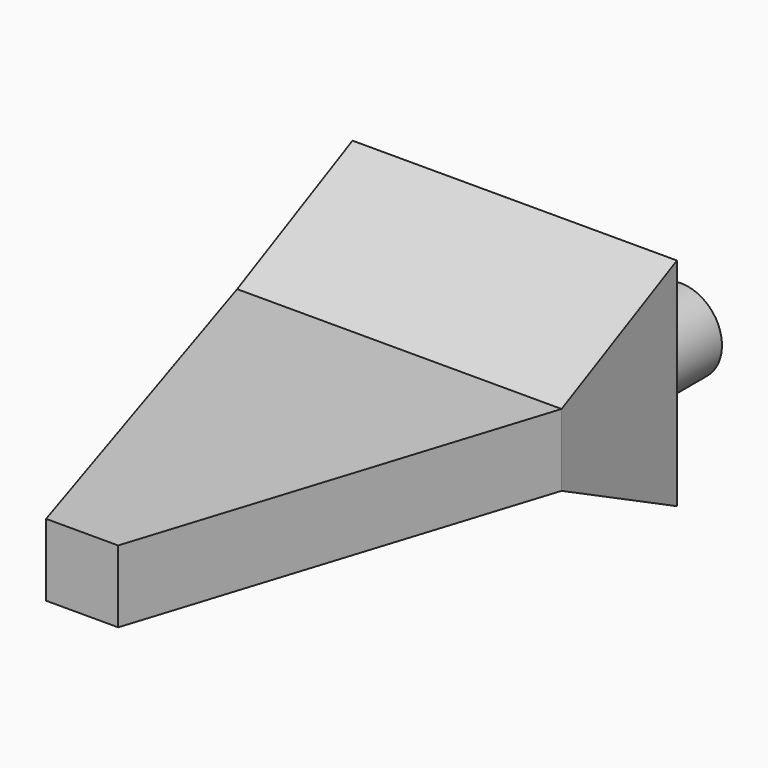
from build123d import *

# Parameters (mm, degrees)
F0_W          = 9
F0_H          = 4
F1_DEPTH      = 2
F2_DEPTH      = 4
F2_DEPTH_BACK = 2
F3_SIZE2      = 3.99999
F3_SIZE       = 1.99999
F4_SIZE2      = 3.99999
F4_SIZE       = 1.99999
F5_R          = 1.15
F6_DEPTH      = 2


# Not quite as in the source:
# - a fillet or chamfer is up to 0.001 mm smaller than in the source, because OpenCascade refuses the exact size


with BuildPart() as f1:
    # F0 (on Top) → F1 (new body)
    with BuildSketch(Plane.XY):
        with Locations((0, 5.5)):
            Rectangle(F0_W, F0_H)
        Polygon((1, -7.5), (4.5, 3.5), (-4.5, 3.5), (-1, -7.5), align=None)
    extrude(amount=F1_DEPTH)

    # F0 (on Top) → F2 (join, two sides)
    with BuildSketch(Plane.XY) as f2_sk:
        with Locations((0, 5.5)):
            Rectangle(F0_W, F0_H)
    extrude(amount=F2_DEPTH)
    extrude(f2_sk.sketch, amount=-F2_DEPTH_BACK)

    # F3 (size 2 and 4 in the source; OpenCascade refuses exactly that, so slightly less here)
    f3_edges = [f1.edges().sort_by_distance(p)[0] for p in [
        (0, 3.5, -2),
    ]]
    f3_side = f1.faces().sort_by_distance((0, 3.5, -1))[0]
    chamfer(f3_edges, length=F3_SIZE, length2=F3_SIZE2, reference=f3_side)

    # F4 (size 2 and 4 in the source; OpenCascade refuses exactly that, so slightly less here)
    f4_edges = [f1.edges().sort_by_distance(p)[0] for p in [
        (0, 3.5, 4),
    ]]
    f4_side = f1.faces().sort_by_distance((0, 3.5, 3))[0]
    chamfer(f4_edges, length=F4_SIZE, length2=F4_SIZE2, reference=f4_side)

    # F5 (on face) → F6 (join)
    with BuildSketch(Plane(origin=(0, 7.5, 0), x_dir=(-1, 0, 0), z_dir=(0, 1, 0))):
        with Locations((-3, 1)):
            Circle(F5_R)
        with Locations((3, 1)):
            Circle(F5_R)
    extrude(amount=F6_DEPTH)


solid = f1.part
